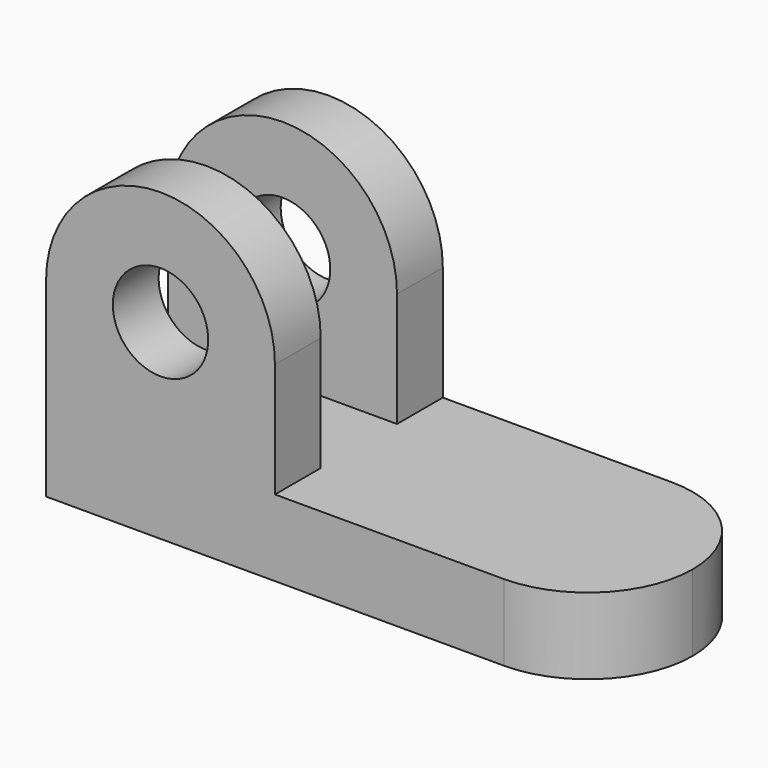
from build123d import *

# Parameters (mm, degrees)
F0_W          = 70
F0_H          = 16
F1_DEPTH      = 22
F1_DEPTH_BACK = 22
F2_DEPTH      = 10
F2_DEPTH_BACK = 10
F3_R          = 21.99999


# Not quite as in the source:
# - a fillet or chamfer is up to 0.001 mm smaller than in the source, because OpenCascade refuses the exact size


with BuildPart() as f1:
    # F0 (on Front) → F1 (new body, two sides)
    with BuildSketch(Plane.XZ) as f1_sk:
        with BuildLine():
            Line((24, 0), (10, 0))
            ThreePointArc((10, 0), (0, -10), (-10, 0))
            Line((-10, 0), (-24, 0))
            ThreePointArc((-24, 0), (-16.9705627485, -16.9705627485), (0, -24))
            ThreePointArc((0, -24), (16.9705627485, -16.9705627485), (24, 0))
        make_face()
        with BuildLine():
            ThreePointArc((-10, 0), (0, 10), (10, 0))
            Line((10, 0), (24, 0))
            ThreePointArc((24, 0), (0, 24), (-24, 0))
            Line((-24, 0), (-10, 0))
        make_face()
        with BuildLine():
            Line((24, -24), (24, 0))
            ThreePointArc((24, 0), (16.9705627485, -16.9705627485), (0, -24))
            Line((0, -24), (24, -24))
        make_face()
        with BuildLine():
            ThreePointArc((0, -24), (-16.9705627485, -16.9705627485), (-24, 0))
            Line((-24, 0), (-24, -24))
            Line((-24, -24), (0, -24))
        make_face()
        Polygon((24, -24), (0, -24), (-24, -24), (-24, -40), (24, -40), align=None)
        with Locations((59, -32)):
            Rectangle(F0_W, F0_H)
    extrude(amount=F1_DEPTH)
    extrude(f1_sk.sketch, amount=-F1_DEPTH_BACK)

    # F0 (on Front) → F2 (cut, two sides)
    with BuildSketch(Plane.XZ) as f2_sk:
        with BuildLine():
            ThreePointArc((-10, 0), (0, 10), (10, 0))
            Line((10, 0), (24, 0))
            ThreePointArc((24, 0), (0, 24), (-24, 0))
            Line((-24, 0), (-10, 0))
        make_face()
        with BuildLine():
            Line((24, -24), (24, 0))
            ThreePointArc((24, 0), (16.9705627485, -16.9705627485), (0, -24))
            Line((0, -24), (24, -24))
        make_face()
        with BuildLine():
            ThreePointArc((0, -24), (-16.9705627485, -16.9705627485), (-24, 0))
            Line((-24, 0), (-24, -24))
            Line((-24, -24), (0, -24))
        make_face()
        with BuildLine():
            Line((24, 0), (10, 0))
            ThreePointArc((10, 0), (0, -10), (-10, 0))
            Line((-10, 0), (-24, 0))
            ThreePointArc((-24, 0), (-16.9705627485, -16.9705627485), (0, -24))
            ThreePointArc((0, -24), (16.9705627485, -16.9705627485), (24, 0))
        make_face()
    extrude(amount=-F2_DEPTH, mode=Mode.SUBTRACT)
    extrude(f2_sk.sketch, amount=F2_DEPTH_BACK, mode=Mode.SUBTRACT)

    # F3 (radius 22 in the source; OpenCascade refuses exactly that, so slightly less here)
    f3_edges = [f1.edges().sort_by_distance(p)[0] for p in [
        (94, -22, -32),
        (94, 22, -32),
    ]]
    fillet(f3_edges, radius=F3_R)


solid = f1.part
